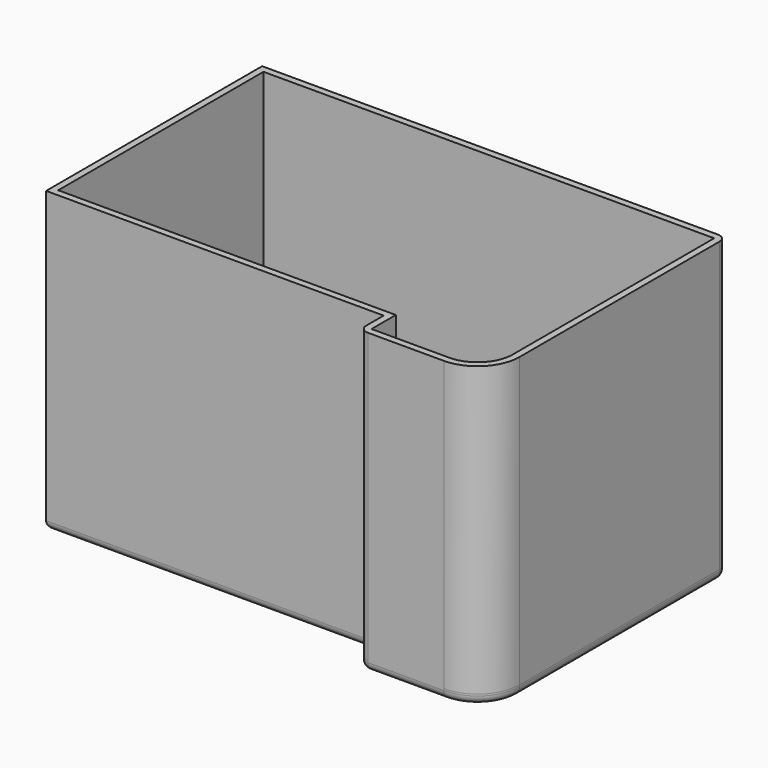
from build123d import *

# Parameters (mm, degrees)
F1_DEPTH     = 1.524
F3_DEPTH     = 43.434
F4_R         = 1.27
F5_T1_DEPTH  = 0.254
F5_T3_DEPTH  = 46.609
F5_S7_W      = 1.27
F5_S7_H      = 1.27
F5_T8_DEPTH  = 1.27
F5_S13_W     = 1.27
F5_S13_H     = 1.27
F5_T14_DEPTH = 1.27


# Not quite as in the source:
# - a fillet or chamfer that OpenCascade refuses, or shapes differently, is made with other operations: its cross-section is extruded or revolved along the edge and cut away or added


with BuildPart() as f1:
    # F0 (on Top) → F1 (new body)
    with BuildSketch(Plane.XY):
        with BuildLine():
            Line((-35.579891, 21.538353), (-35.579891, -17.323647))
            ThreePointArc((-35.579891, -17.323647), (-33.720019, -21.813775), (-29.229891, -23.673647))
            Line((-29.229891, -23.673647), (-16.529891, -23.673647))
            Line((-16.529891, -23.673647), (-16.529891, -19.101647))
            Line((-16.529891, -19.101647), (34.270109, -19.101647))
            Line((34.270109, -19.101647), (34.270109, 21.538353))
            Line((34.270109, 21.538353), (-35.579891, 21.538353))
        make_face()
    extrude(amount=F1_DEPTH)

    # F2 (on face) → F3 (join)
    with BuildSketch(Plane.XY.offset(1.524)):
        with BuildLine():
            Line((-35.57989, 21.538353), (-35.57989, -17.323647))
            ThreePointArc((-35.57989, -17.323647), (-33.720018, -21.813775), (-29.22989, -23.673647))
            Line((-29.22989, -23.673647), (-16.52989, -23.673647))
            Line((-16.52989, -23.673647), (-16.52989, -19.101647))
            Line((-16.52989, -19.101647), (34.27011, -19.101647))
            Line((34.27011, -19.101647), (34.27011, 21.538353))
            Line((34.27011, 21.538353), (-35.57989, 21.538353))
        make_face()
        with BuildLine():
            Line((33.25411, -18.085647), (-17.54589, -18.085647))
            Line((-17.54589, -18.085647), (-17.54589, -22.657647))
            Line((-17.54589, -22.657647), (-29.22989, -22.657647))
            ThreePointArc((-29.22989, -22.657647), (-33.001598, -21.095355), (-34.56389, -17.323647))
            Line((-34.56389, -17.323647), (-34.56389, 20.522353))
            Line((-34.56389, 20.522353), (33.25411, 20.522353))
            Line((33.25411, 20.522353), (33.25411, -18.085647))
        make_face(mode=Mode.SUBTRACT)
    extrude(amount=F3_DEPTH)

    # F4
    f4_edges = [f1.edges().sort_by_distance(p)[0] for p in [
        (-0.654891, 21.538353, 0),
        (-35.579891, 2.107353, 0),
        (-33.720019, -21.813775, 0),
        (-22.879891, -23.673647, 0),
        (-16.529891, -21.387647, 0),
        (8.870109, -19.101647, 0),
        (34.270109, 1.218353, 0),
    ]]
    fillet(f4_edges, radius=F4_R)

    # F5: fillet of radius 1.27 on 4 edges, made by hand

    # F5_s2 → F5_t1 (cut)
    with BuildSketch(Plane.XY.offset(1.27)):
        with BuildLine():
            ThreePointArc((-17.799891, -23.673647), (-16.901866, -23.301673), (-16.529891, -22.403647))
            Line((-16.529891, -22.403647), (-16.529891, -23.673647))
            Line((-16.529891, -23.673647), (-17.799891, -23.673647))
        make_face()
        with BuildLine():
            ThreePointArc((-34.309891, 21.538353), (-35.207917, 21.166379), (-35.579891, 20.268353))
            Line((-35.579891, 20.268353), (-35.579891, 21.538353))
            Line((-35.579891, 21.538353), (-34.309891, 21.538353))
        make_face()
    extrude(amount=F5_T1_DEPTH, mode=Mode.SUBTRACT)

    # F5_s4 → F5_t3 (cut)
    with BuildSketch(Plane.XY.offset(1.524)):
        with BuildLine():
            ThreePointArc((-17.79989, -23.673647), (-16.901864, -23.301673), (-16.52989, -22.403647))
            Line((-16.52989, -22.403647), (-16.52989, -23.673647))
            Line((-16.52989, -23.673647), (-17.79989, -23.673647))
        make_face()
        with BuildLine():
            ThreePointArc((-34.30989, 21.538353), (-35.207916, 21.166379), (-35.57989, 20.268353))
            Line((-35.57989, 20.268353), (-35.57989, 21.538353))
            Line((-35.57989, 21.538353), (-34.30989, 21.538353))
        make_face()
    extrude(amount=F5_T3_DEPTH, mode=Mode.SUBTRACT)


with BuildPart() as f5_tool6:
    # F5_s7 → F5_t8 (new body)
    with BuildSketch(Plane.XZ.offset(-20.268353)):
        with Locations((-34.944891, 0.635)):
            Rectangle(F5_S7_W, F5_S7_H)
    extrude(amount=-F5_T8_DEPTH)

    # F5_s9 → F5_t10 (revolve, cut)
    with BuildSketch(Plane(origin=(-34.309891, 20.268353, 1.27), x_dir=(0.707107, 0, 0.707107), z_dir=(-0.707107, 0, 0.707107))):
        with BuildLine():
            ThreePointArc((0, -1.27), (1.27, 0), (0, 1.27))
            Line((0, 1.27), (0, -1.27))
        make_face()
    revolve(axis=Axis((-34.309891, 20.268353, 1.27), (0, 1, 0)), mode=Mode.SUBTRACT)


with BuildPart() as f1_1:
    add(f1.part)

    # F5_t5: cut F5_tool6
    add(f5_tool6.part, mode=Mode.SUBTRACT)


with BuildPart() as f5_tool12:
    # F5_s13 → F5_t14 (new body)
    with BuildSketch(Plane.XZ.offset(22.403647)):
        with Locations((-17.164891, 0.635)):
            Rectangle(F5_S13_W, F5_S13_H)
    extrude(amount=F5_T14_DEPTH)

    # F5_s15 → F5_t16 (revolve, cut)
    with BuildSketch(Plane(origin=(-17.799891, -22.403647, 1.27), x_dir=(-0.707107, 0, 0.707107), z_dir=(0.707107, 0, 0.707107))):
        with BuildLine():
            ThreePointArc((0, -1.27), (1.27, 0), (0, 1.27))
            Line((0, 1.27), (0, -1.27))
        make_face()
    revolve(axis=Axis((-17.799891, -22.403647, 1.27), (0, -1, 0)), mode=Mode.SUBTRACT)


with BuildPart() as f1_2:
    add(f1_1.part)

    # F5_t11: cut F5_tool12
    add(f5_tool12.part, mode=Mode.SUBTRACT)


with BuildPart() as f6_1:
    # F6: instance of F1
    add(f1_2.part.mirror(Plane(origin=(34.270109, 1.218353, 1.397), x_dir=(0, 1, 0), z_dir=(1, 0, 0))))


solid = f6_1.part
